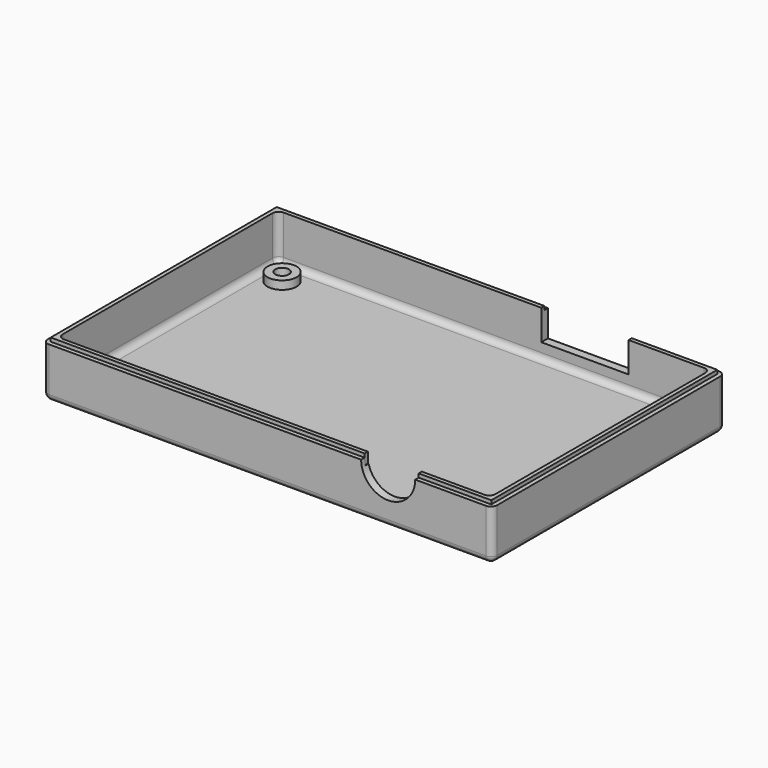
from build123d import *

# Parameters (mm, degrees)
F0_W           = 108
F0_H           = 70
F0_W_2         = 105.9
F0_H_2         = 67.9
F0_W_3         = 104
F0_H_3         = 66
F0_R           = 3
F1_DEPTH       = 2
F2_DEPTH       = 10.99
F3_DEPTH       = 10.1
F4_R           = 3.5
F5_DEPTH       = 2
F7_D           = 3.302
F7_CSINK_D     = 6.477
F7_CSINK_ANGLE = 82
F8_W           = 21
F8_H           = 6.4
F9_DEPTH       = 2.5
F10_W          = 13
F10_H          = 0.95
F11_DEPTH      = 2.5
F13_DEPTH      = 2.5
F14_R          = 1.5
F15_R          = 1.5
F16_W          = 21
F16_H          = 0.89
F17_DEPTH      = 2.5


# Not quite as in the source:
# - a feature names something its author has since deleted; it is built from what else it names


with BuildPart() as f1:
    # F0 (on Top) → F1 (new body)
    with BuildSketch(Plane.XY):
        with Locations((9.6408709802, -2.0854342729)):
            Rectangle(F0_W, F0_H)
        with Locations((9.6408709802, -2.0854342729)):
            Rectangle(F0_W_2, F0_H_2, mode=Mode.SUBTRACT)
        with Locations((9.6408709802, -2.0854342729)):
            Rectangle(F0_W_2, F0_H_2)
        with Locations((9.6408709802, -2.0854342729)):
            Rectangle(F0_W_3, F0_H_3, mode=Mode.SUBTRACT)
        with Locations((9.6408709802, -2.0854342729)):
            Rectangle(F0_W_3, F0_H_3)
        with Locations((-36.8591290198, -29.5854342729)):
            Circle(F0_R, mode=Mode.SUBTRACT)
        with Locations((54.9200624228, -29.5854342729)):
            Circle(F0_R, mode=Mode.SUBTRACT)
        with Locations((-36.8591290198, 25.4145657271)):
            Circle(F0_R, mode=Mode.SUBTRACT)
        with Locations((57.1408709802, 25.4145657271)):
            Circle(F0_R, mode=Mode.SUBTRACT)
        with Locations((-36.8591290198, -29.5854342729)):
            Circle(F0_R)
        with Locations((54.9200624228, -29.5854342729)):
            Circle(F0_R)
        with Locations((-36.8591290198, 25.4145657271)):
            Circle(F0_R)
        with Locations((57.1408709802, 25.4145657271)):
            Circle(F0_R)
    extrude(amount=-F1_DEPTH)

    # F0 (on Top) → F2 (join)
    with BuildSketch(Plane.XY):
        with Locations((9.6408709802, -2.0854342729)):
            Rectangle(F0_W_2, F0_H_2)
        with Locations((9.6408709802, -2.0854342729)):
            Rectangle(F0_W_3, F0_H_3, mode=Mode.SUBTRACT)
    extrude(amount=F2_DEPTH)

    # F0 (on Top) → F3 (join)
    with BuildSketch(Plane.XY):
        with Locations((9.6408709802, -2.0854342729)):
            Rectangle(F0_W, F0_H)
        with Locations((9.6408709802, -2.0854342729)):
            Rectangle(F0_W_2, F0_H_2, mode=Mode.SUBTRACT)
    extrude(amount=F3_DEPTH)

    # F4 (on face) → F5 (join)
    with BuildSketch(Plane.XY):
        with Locations((-36.8591290198, 25.4145657271)):
            Circle(F4_R)
        with Locations((56.1408709802, 25.4145657271)):
            Circle(F4_R)
        with Locations((56.1408709802, -29.5854342729)):
            Circle(F4_R)
        with Locations((-36.8591290198, -29.5854342729)):
            Circle(F4_R)
    extrude(amount=F5_DEPTH)

    # F7 (through all)
    with Locations(Plane(origin=(0, 0, -2), x_dir=(1, 0, 0), z_dir=(0, 0, -1))):
        with Locations((-36.8591290198, 29.5854342729), (56.1408709802, 29.5854342729), (56.1408709802, -25.4145657271), (-36.8591290198, -25.4145657271)):
            CounterSinkHole(F7_D / 2, F7_CSINK_D / 2, counter_sink_angle=F7_CSINK_ANGLE)

    # F8 (on face) → F9 (cut)
    with BuildSketch(Plane(origin=(0, 32.9145657271, 0), x_dir=(-1, 0, 0), z_dir=(0, 1, 0))):
        with Locations((-31.5408709802, 6.9)):
            Rectangle(F8_W, F8_H)
    extrude(amount=-F9_DEPTH, mode=Mode.SUBTRACT)

    # F10 (on face) → F11 (cut)
    with BuildSketch(Plane.XY.offset(10.99)):
        with Locations((38.6408709802, -35.5604342729)):
            Rectangle(F10_W, F10_H)
    extrude(amount=-F11_DEPTH, mode=Mode.SUBTRACT)

    # F12 (on face) → F13 (cut)
    with BuildSketch(Plane.XZ.offset(37.0854342729)):
        with BuildLine():
            ThreePointArc((32.1408709802, 10.1), (38.6408709802, 3.6), (45.1408709802, 10.1))
            Line((45.1408709802, 10.1), (32.1408709802, 10.1))
        make_face()
    extrude(amount=-F13_DEPTH, mode=Mode.SUBTRACT)

    # F14
    f14_edges = [f1.edges().sort_by_distance(p)[0] for p in [
        (63.640871, -37.085434, 4.05),
        (63.640871, -2.085434, -2),
        (63.640871, 32.914566, 4.05),
        (9.640871, 32.914566, -2),
        (-44.359129, 32.914566, 4.05),
        (-44.359129, -37.085434, 4.05),
        (-44.359129, -2.085434, -2),
        (9.640871, -37.085434, -2),
    ]]
    fillet(f14_edges, radius=F14_R)

    # F15
    f15_edges = [f1.edges().sort_by_distance(p)[0] for p in [
        (9.640871, 30.914566, 0),
        (-42.359129, 30.914566, 5.495),
        (-42.359129, -2.085434, 0),
        (9.640871, -35.085434, 0),
        (-42.359129, -35.085434, 5.495),
        (61.640871, 30.914566, 5.495),
        (61.640871, -2.085434, 0),
        (61.640871, -35.085434, 5.495),
    ]]
    fillet(f15_edges, radius=F15_R)

    # F16 (on face) → F17 (cut)
    with BuildSketch(Plane(origin=(0, 31.8645657271, 0), x_dir=(-1, 0, 0), z_dir=(0, 1, 0))):
        with Locations((-31.5408709802, 10.545)):
            Rectangle(F16_W, F16_H)
    extrude(amount=-F17_DEPTH, mode=Mode.SUBTRACT)


solid = f1.part
